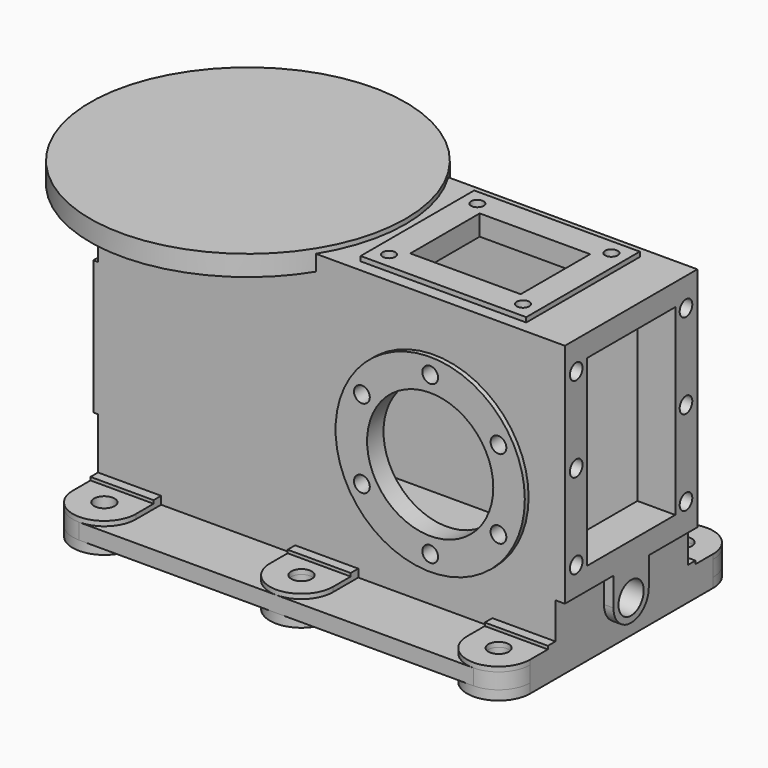
from build123d import *

# Parameters (mm, degrees)
F1_R           = 6.5
F2_DEPTH       = 10
F3_R           = 6.5
F4_DEPTH       = 6
F4_DEPTH_BACK  = 15
F5_W           = 396.017335
F5_H           = 57.627901
F5_W_2         = 411.018034
F5_H_2         = 80.782652
F6_DEPTH       = 2
F7_W           = 290
F7_H           = 172
F8_DEPTH       = 52.5
F8_DEPTH_BACK  = 52.5
F9_W           = 191
F9_H           = 162
F10_DEPTH      = 42.5
F10_DEPTH_BACK = 42.5
F12_DEPTH      = 6
F13_W          = 70
F13_H          = 116
F14_DEPTH      = 24
F16_D          = 20
F16_DEPTH      = 40
F16_TIP        = 6.008606
F18_D          = 10
F18_DEPTH      = 15
F18_TIP        = 3.004303
F19_W          = 105
F19_H          = 90
F19_W_2        = 70
F19_H_2        = 55
F20_DEPTH      = 3
F21_DEPTH      = 10
F22_R          = 4
F23_DEPTH      = 25
F24_W          = 105
F24_H          = 85
F25_DEPTH      = 3
F26_R          = 32
F27_DEPTH      = 84
F29_D          = 10
F29_DEPTH      = 15
F29_TIP        = 3.004303
F30_R          = 60
F31_DEPTH      = 3
F32_R          = 40
F33_DEPTH      = 13
F35_D          = 10
F35_DEPTH      = 15
F35_TIP        = 3.004303
F36_R          = 100
F37_DEPTH      = 13


with BuildPart() as f2:
    # F1 (on offset) → F2 (new body)
    with BuildSketch(Plane.XY.offset(-90)):
        with BuildLine():
            Line((77, -72.5), (77, 72.5))
            ThreePointArc((77, 72.5), (71.142136, 86.642136), (57, 92.5))
            ThreePointArc((57, 92.5), (42.857864, 86.642136), (37, 72.5))
            Line((37, 72.5), (37, -72.5))
            ThreePointArc((37, -72.5), (42.857864, -86.642136), (57, -92.5))
            ThreePointArc((57, -92.5), (71.142136, -86.642136), (77, -72.5))
        make_face()
        with Locations((57, -72.5)):
            Circle(F1_R, mode=Mode.SUBTRACT)
        with Locations((57, 72.5)):
            Circle(F1_R, mode=Mode.SUBTRACT)
        with BuildLine():
            ThreePointArc((37, 72.5), (42.857864, 86.642136), (57, 92.5))
            Line((57, 92.5), (-68, 92.5))
            ThreePointArc((-68, 92.5), (-53.857864, 86.642136), (-48, 72.5))
            Line((-48, 72.5), (-48, -72.5))
            ThreePointArc((-48, -72.5), (-53.857864, -86.642136), (-68, -92.5))
            Line((-68, -92.5), (57, -92.5))
            ThreePointArc((57, -92.5), (42.857864, -86.642136), (37, -72.5))
            Line((37, -72.5), (37, 72.5))
        make_face()
        with BuildLine():
            ThreePointArc((-48, 72.5), (-53.857864, 86.642136), (-68, 92.5))
            ThreePointArc((-68, 92.5), (-82.142136, 86.642136), (-88, 72.5))
            Line((-88, 72.5), (-88, -72.5))
            ThreePointArc((-88, -72.5), (-82.142136, -86.642136), (-68, -92.5))
            ThreePointArc((-68, -92.5), (-53.857864, -86.642136), (-48, -72.5))
            Line((-48, -72.5), (-48, 72.5))
        make_face()
        with Locations((-68, -72.5)):
            Circle(F1_R, mode=Mode.SUBTRACT)
        with Locations((-68, 72.5)):
            Circle(F1_R, mode=Mode.SUBTRACT)
        with BuildLine():
            ThreePointArc((-88, 72.5), (-82.142136, 86.642136), (-68, 92.5))
            Line((-68, 92.5), (-193, 92.5))
            ThreePointArc((-193, 92.5), (-178.857864, 86.642136), (-173, 72.5))
            Line((-173, 72.5), (-173, -72.5))
            ThreePointArc((-173, -72.5), (-178.857864, -86.642136), (-193, -92.5))
            Line((-193, -92.5), (-68, -92.5))
            ThreePointArc((-68, -92.5), (-82.142136, -86.642136), (-88, -72.5))
            Line((-88, -72.5), (-88, 72.5))
        make_face()
        with BuildLine():
            ThreePointArc((-173, 72.5), (-178.857864, 86.642136), (-193, 92.5))
            ThreePointArc((-193, 92.5), (-207.142136, 86.642136), (-213, 72.5))
            Line((-213, 72.5), (-213, -72.5))
            ThreePointArc((-213, -72.5), (-207.142136, -86.642136), (-193, -92.5))
            ThreePointArc((-193, -92.5), (-178.857864, -86.642136), (-173, -72.5))
            Line((-173, -72.5), (-173, 72.5))
        make_face()
        with Locations((-193, -72.5)):
            Circle(F1_R, mode=Mode.SUBTRACT)
        with Locations((-193, 72.5)):
            Circle(F1_R, mode=Mode.SUBTRACT)
    extrude(amount=F2_DEPTH)

    # F3 (on face) → F4 (join, two sides)
    with BuildSketch(Plane(origin=(0, 0, -90), x_dir=(1, 0, 0), z_dir=(0, 0, -1))) as f4_sk:
        with BuildLine():
            Line((77, -72.5), (77, 72.5))
            ThreePointArc((77, 72.5), (57, 92.5), (37, 72.5))
            Line((37, 72.5), (37, -72.5))
            ThreePointArc((37, -72.5), (57, -92.5), (77, -72.5))
        make_face()
        with Locations((57, -72.5)):
            Circle(F3_R, mode=Mode.SUBTRACT)
        with Locations((57, 72.5)):
            Circle(F3_R, mode=Mode.SUBTRACT)
        with BuildLine():
            Line((-48, -72.5), (-48, 72.5))
            ThreePointArc((-48, 72.5), (-68, 92.5), (-88, 72.5))
            Line((-88, 72.5), (-88, -72.5))
            ThreePointArc((-88, -72.5), (-68, -92.5), (-48, -72.5))
        make_face()
        with Locations((-68, -72.5)):
            Circle(F3_R, mode=Mode.SUBTRACT)
        with Locations((-68, 72.5)):
            Circle(F3_R, mode=Mode.SUBTRACT)
        with BuildLine():
            Line((-173, -72.5), (-173, 72.5))
            ThreePointArc((-173, 72.5), (-193, 92.5), (-213, 72.5))
            Line((-213, 72.5), (-213, -72.5))
            ThreePointArc((-213, -72.5), (-193, -92.5), (-173, -72.5))
        make_face()
        with Locations((-193, -72.5)):
            Circle(F3_R, mode=Mode.SUBTRACT)
        with Locations((-193, 72.5)):
            Circle(F3_R, mode=Mode.SUBTRACT)
    extrude(amount=F4_DEPTH)
    extrude(f4_sk.sketch, amount=-F4_DEPTH_BACK)

    # F5 (on face) → F6 (cut)
    with BuildSketch(Plane.XY.offset(-75)):
        with Locations((-82.299638, 87.313951)):
            Rectangle(F5_W, F5_H)
        with Locations((-95.071438, -98.891326)):
            Rectangle(F5_W_2, F5_H_2)
    extrude(amount=-F6_DEPTH, mode=Mode.SUBTRACT)

    # F7 (on Front) → F8 (join, two sides)
    with BuildSketch(Plane.XZ) as f8_sk:
        with Locations((-68, 6)):
            Rectangle(F7_W, F7_H)
    extrude(amount=F8_DEPTH)
    extrude(f8_sk.sketch, amount=-F8_DEPTH_BACK)

    # F9 (on Front) → F10 (cut, two sides)
    with BuildSketch(Plane.XZ) as f10_sk:
        with Locations((-36.5, 1)):
            Rectangle(F9_W, F9_H)
    extrude(amount=-F10_DEPTH, mode=Mode.SUBTRACT)
    extrude(f10_sk.sketch, amount=F10_DEPTH_BACK, mode=Mode.SUBTRACT)

    # F11 (on face) → F12 (join)
    with BuildSketch(Plane.YZ.offset(77)):
        with BuildLine():
            Line((52.5, 92), (-52.5, 92))
            Line((-52.5, 92), (-52.5, -52))
            Line((-52.5, -52), (-14, -52))
            Line((-14, -52), (-14, -70))
            ThreePointArc((-14, -70), (0, -84), (14, -70))
            Line((14, -70), (14, -52))
            Line((14, -52), (52.5, -52))
            Line((52.5, -52), (52.5, 92))
        make_face()
    extrude(amount=F12_DEPTH)

    # F13 (on face) → F14 (cut, through all)
    with BuildSketch(Plane.YZ.offset(83)):
        with Locations((0, 20)):
            Rectangle(F13_W, F13_H)
    extrude(amount=-F14_DEPTH, mode=Mode.SUBTRACT)

    # F16
    with Locations(Plane.YZ.offset(83)):
        with Locations((0, -70)):
            Hole(F16_D / 2, depth=F16_DEPTH)
            with Locations((0, 0, -(F16_DEPTH + F16_TIP / 2))):  # 118° drill point
                Cone(0, F16_D / 2, F16_TIP, mode=Mode.SUBTRACT)

    # F18
    with Locations(Plane.YZ.offset(83)):
        with Locations((-43.5, 74), (-43.5, 20), (-43.5, -34), (43.5, 74), (43.5, 20), (43.5, -34)):
            Hole(F18_D / 2, depth=F18_DEPTH)
            with Locations((0, 0, -(F18_DEPTH + F18_TIP / 2))):  # 118° drill point
                Cone(0, F18_D / 2, F18_TIP, mode=Mode.SUBTRACT)

    # F19 (on face) → F20 (join)
    with BuildSketch(Plane.XY.offset(92)):
        Rectangle(F19_W, F19_H)
        Rectangle(F19_W_2, F19_H_2, mode=Mode.SUBTRACT)
    extrude(amount=F20_DEPTH)

    # F21 (cut, through all): a face of the model
    f21_faces = [f2.faces().sort_by_distance(p)[0] for p in [
        (0, 0, 92),
    ]]
    extrude(f21_faces, amount=-F21_DEPTH, mode=Mode.SUBTRACT)

    # F22 (on face) → F23 (cut)
    with BuildSketch(Plane.XY.offset(95)):
        with Locations((-42.5, 35)):
            Circle(F22_R)
        with Locations((42.5, 35)):
            Circle(F22_R)
        with Locations((42.5, -35)):
            Circle(F22_R)
        with Locations((-42.5, -35)):
            Circle(F22_R)
    extrude(amount=-F23_DEPTH, mode=Mode.SUBTRACT)

    # F24 (on face) → F25 (join)
    with BuildSketch(Plane(origin=(-213, 0, 0), x_dir=(0, -1, 0), z_dir=(-1, 0, 0))):
        Rectangle(F24_W, F24_H)
    extrude(amount=F25_DEPTH)

    # F26 (on face) → F27 (cut, through all)
    with BuildSketch(Plane(origin=(-216, 0, 0), x_dir=(0, -1, 0), z_dir=(-1, 0, 0))):
        Circle(F26_R)
    extrude(amount=-F27_DEPTH, mode=Mode.SUBTRACT)

    # F29
    with Locations(Plane(origin=(-216, 0, 0), x_dir=(0, -1, 0), z_dir=(-1, 0, 0))):
        with Locations((-42.5, 26), (42.5, -26), (-42.5, -26), (42.5, 26)):
            Hole(F29_D / 2, depth=F29_DEPTH)
            with Locations((0, 0, -(F29_DEPTH + F29_TIP / 2))):  # 118° drill point
                Cone(0, F29_D / 2, F29_TIP, mode=Mode.SUBTRACT)

    # F30 (on face) → F31 (join)
    with BuildSketch(Plane.XZ.offset(52.5)):
        Circle(F30_R)
    extrude(amount=F31_DEPTH)

    # F32 (on face) → F33 (cut, through all)
    with BuildSketch(Plane.XZ.offset(55.5)):
        Circle(F32_R)
    extrude(amount=-F33_DEPTH, mode=Mode.SUBTRACT)

    # F35
    with Locations(Plane.XZ.offset(55.5)):
        with Locations((0, 50), (43.30127, 25), (43.30127, -25), (0, -50), (-43.30127, -25), (-43.30127, 25)):
            Hole(F35_D / 2, depth=F35_DEPTH)
            with Locations((0, 0, -(F35_DEPTH + F35_TIP / 2))):  # 118° drill point
                Cone(0, F35_D / 2, F35_TIP, mode=Mode.SUBTRACT)


with BuildPart() as f37:
    # F36 (on face) → F37 (new body)
    with BuildSketch(Plane.XY.offset(95)):
        with Locations((-160, 0)):
            Circle(F36_R)
    extrude(amount=-F37_DEPTH)


solid = Compound([f2.part, f37.part])
